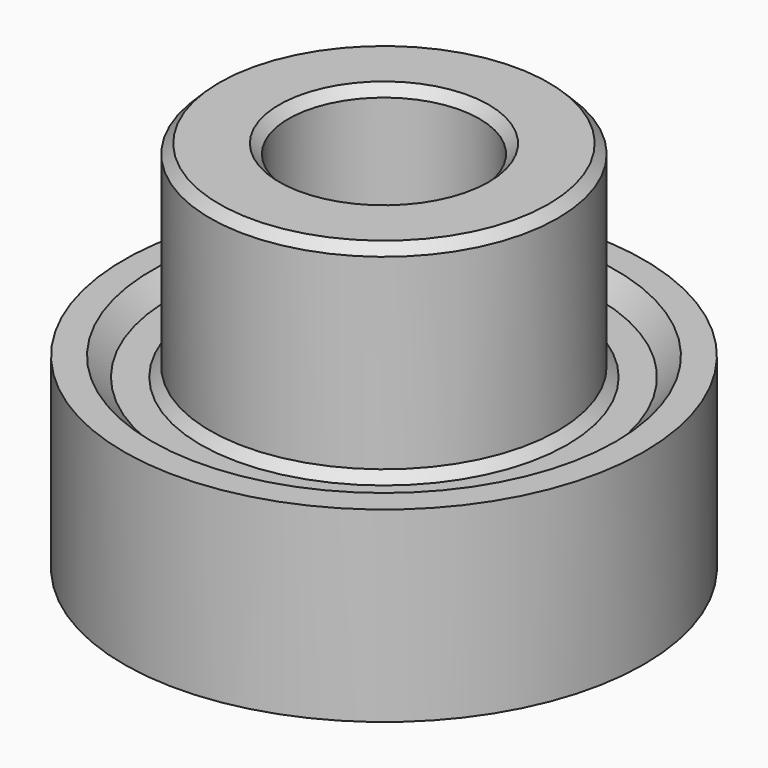
from build123d import *

# Parameters (mm, degrees)
F0_R     = 13.9
F0_R_2   = 12.4
F1_DEPTH = 10
F0_R_3   = 9.3
F2_DEPTH = 9
F0_R_4   = 5.1
F3_DEPTH = 20
F4_SIZE  = 0.5
F5_SIZE  = 0.99999


# Not quite as in the source:
# - a fillet or chamfer is up to 0.001 mm smaller than in the source, because OpenCascade refuses the exact size


with BuildPart() as f1:
    # F0 (on Top) → F1 (new body)
    with BuildSketch(Plane.XY):
        Circle(F0_R)
        Circle(F0_R_2, mode=Mode.SUBTRACT)
    extrude(amount=F1_DEPTH)

    # F0 (on Top) → F2 (join)
    with BuildSketch(Plane.XY):
        Circle(F0_R)
        Circle(F0_R_2, mode=Mode.SUBTRACT)
        Circle(F0_R_2)
        Circle(F0_R_3, mode=Mode.SUBTRACT)
    extrude(amount=F2_DEPTH)

    # F0 (on Top) → F3 (join)
    with BuildSketch(Plane.XY):
        Circle(F0_R_3)
        Circle(F0_R_4, mode=Mode.SUBTRACT)
    extrude(amount=F3_DEPTH)

    # F4
    f4_edges = [f1.edges().sort_by_distance(p)[0] for p in [
        (-5.1, 0, 20),
        (-9.3, 0, 20),
        (-9.3, 0, 9),
        (-5.1, 0, 0),
    ]]
    chamfer(f4_edges, length=F4_SIZE)

    # F5 (size 1 in the source; OpenCascade refuses exactly that, so slightly less here)
    f5_edges = [f1.edges().sort_by_distance(p)[0] for p in [
        (-12.4, 0, 9),
    ]]
    chamfer(f5_edges, length=F5_SIZE)


solid = f1.part
